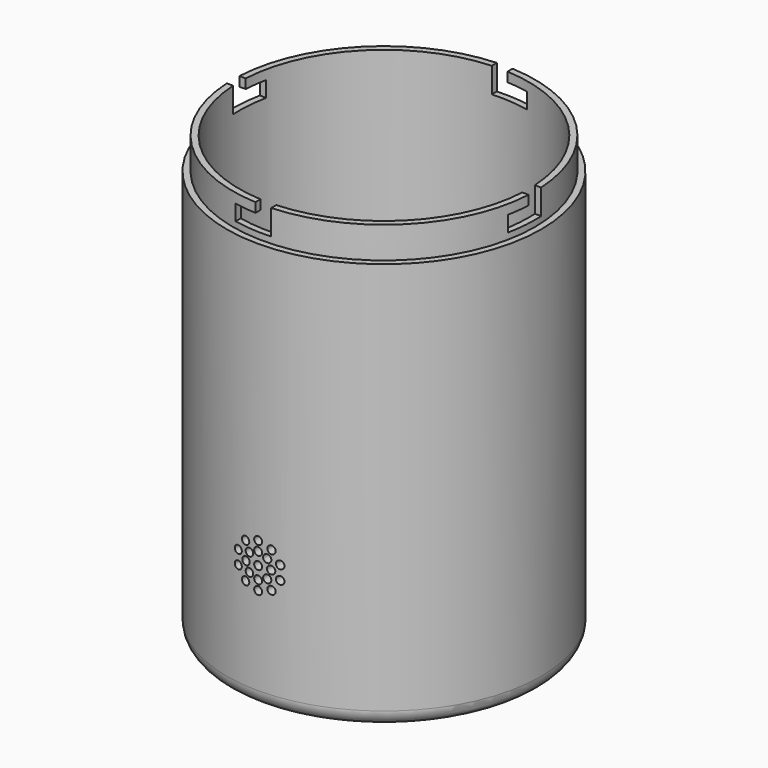
from build123d import *

# Parameters (mm, degrees)
F0_R            = 50
F0_R_2          = 2.5
F1_DEPTH        = 130
F2_T            = -4
F3_R            = 5
F4_DEPTH        = 130.001
F5_R            = 48
F5_R_2          = 46
F6_DEPTH        = 10
F7_W            = 7
F7_H            = 5
F8_DEPTH        = 50.0010001
F8_COPIES_COUNT = 4
F9_R            = 1.25
F10_DEPTH       = 50.001
F10_DEPTH_BACK  = 50.0010001


# Not quite as in the source:
# - a pattern or mirror of a feature is missing from the dataset's text; its kind, count and spacing are read off the source's solid


with BuildPart() as f1:
    # F0 (on Top) → F1 (new body)
    with BuildSketch(Plane.XY):
        Circle(F0_R)
        with Locations((-2.1631189606, -6.6573956141)):
            Circle(F0_R_2, mode=Mode.SUBTRACT)
        with Locations((5.6631189606, -4.114496766)):
            Circle(F0_R_2, mode=Mode.SUBTRACT)
        with Locations((-7, 0)):
            Circle(F0_R_2, mode=Mode.SUBTRACT)
        with Locations((-2.1631189606, 6.6573956141)):
            Circle(F0_R_2, mode=Mode.SUBTRACT)
        Circle(F0_R_2, mode=Mode.SUBTRACT)
        with Locations((5.6631189606, 4.114496766)):
            Circle(F0_R_2, mode=Mode.SUBTRACT)
        with Locations((-2.1631189606, -6.6573956141)):
            Circle(F0_R_2)
        with Locations((5.6631189606, -4.114496766)):
            Circle(F0_R_2)
        with Locations((5.6631189606, 4.114496766)):
            Circle(F0_R_2)
        Circle(F0_R_2)
        with Locations((-7, 0)):
            Circle(F0_R_2)
        with Locations((-2.1631189606, 6.6573956141)):
            Circle(F0_R_2)
    extrude(amount=F1_DEPTH)

    # F2
    f2_openings = [f1.faces().sort_by_distance(p)[0] for p in [
        (0, 0, 130),
    ]]
    offset(amount=F2_T, openings=f2_openings)

    # F3
    f3_edges = [f1.edges().sort_by_distance(p)[0] for p in [
        (-50, 0, 0),
    ]]
    fillet(f3_edges, radius=F3_R)

    # F0 (on Top) → F4 (cut, through all)
    with BuildSketch(Plane.XY):
        with Locations((5.6631189606, -4.114496766)):
            Circle(F0_R_2)
        with Locations((-2.1631189606, -6.6573956141)):
            Circle(F0_R_2)
        Circle(F0_R_2)
        with Locations((-2.1631189606, 6.6573956141)):
            Circle(F0_R_2)
        with Locations((5.6631189606, 4.114496766)):
            Circle(F0_R_2)
        with Locations((-7, 0)):
            Circle(F0_R_2)
    extrude(amount=F4_DEPTH, mode=Mode.SUBTRACT)

    # F5 (on face) → F6 (join)
    with BuildSketch(Plane.XY.offset(130)):
        Circle(F5_R)
        Circle(F5_R_2, mode=Mode.SUBTRACT)
    extrude(amount=F6_DEPTH)

    # F7 (on Front) → F8 (cut, through all)
    with BuildSketch(Plane.XZ):
        with Locations((-6, 134.5)):
            Rectangle(F7_W, F7_H)
        Polygon((2.5, 140), (-2.5, 140), (-2.5, 137), (-2.5, 132), (2.5, 132), align=None)
    f8 = extrude(amount=F8_DEPTH, mode=Mode.SUBTRACT)

    # F8_copies: F8 ×4 about axis
    f8_copies_axis = Axis((0, 0, 0), (0, 0, 1))
    for i in range(1, F8_COPIES_COUNT):
        add(f8.rotate(f8_copies_axis, i * 360 / F8_COPIES_COUNT), mode=Mode.SUBTRACT)

    # F9 (on Front) → F10 (cut, two sides)
    with BuildSketch(Plane.XZ) as f10_sk:
        with Locations((0, 40)):
            Circle(F9_R)
        with Locations((0, 44)):
            Circle(F9_R)
        with Locations((-2.8284271247, 42.8284271247)):
            Circle(F9_R)
        with Locations((-4, 40)):
            Circle(F9_R)
        with Locations((-2.8284271247, 37.1715728753)):
            Circle(F9_R)
        with Locations((0, 36)):
            Circle(F9_R)
        with Locations((2.8284271247, 37.1715728753)):
            Circle(F9_R)
        with Locations((4, 40)):
            Circle(F9_R)
        with Locations((2.8284271247, 42.8284271247)):
            Circle(F9_R)
        with Locations((0, 47)):
            Circle(F9_R)
        with Locations((-4.114496766, 45.6631189606)):
            Circle(F9_R)
        with Locations((-6.6573956141, 42.1631189606)):
            Circle(F9_R)
        with Locations((-6.6573956141, 37.8368810394)):
            Circle(F9_R)
        with Locations((-4.114496766, 34.3368810394)):
            Circle(F9_R)
        with Locations((0, 33)):
            Circle(F9_R)
        with Locations((4.114496766, 34.3368810394)):
            Circle(F9_R)
        with Locations((6.6573956141, 37.8368810394)):
            Circle(F9_R)
        with Locations((6.6573956141, 42.1631189606)):
            Circle(F9_R)
        with Locations((4.114496766, 45.6631189606)):
            Circle(F9_R)
    extrude(amount=-F10_DEPTH, mode=Mode.SUBTRACT)
    extrude(f10_sk.sketch, amount=F10_DEPTH_BACK, mode=Mode.SUBTRACT)


solid = f1.part
